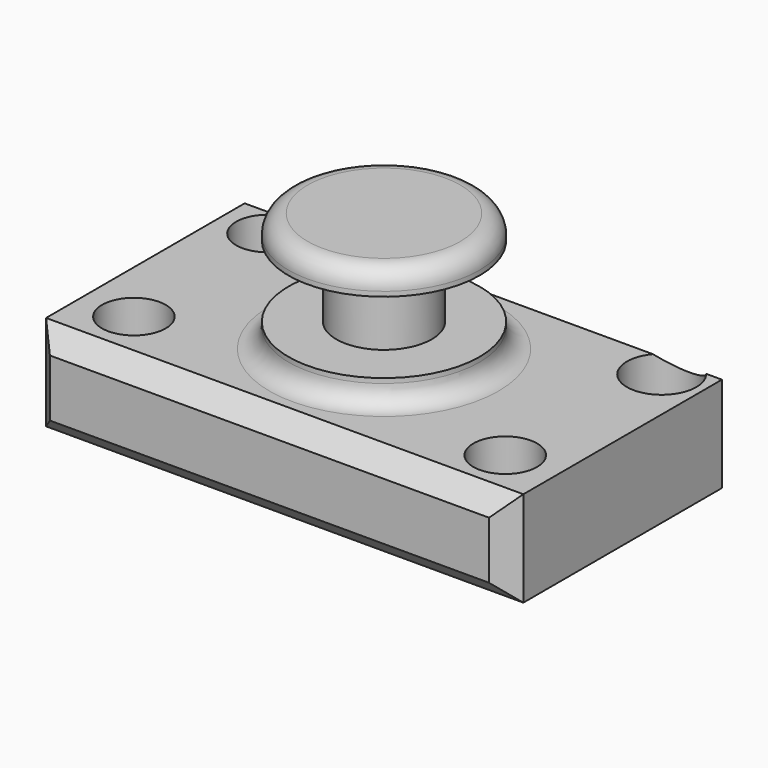
from build123d import *

# Parameters (mm, degrees)
F0_W         = 127
F0_H         = 76.2
F1_DEPTH     = 25.4
F2_R         = 8.4769821521
F2_R_2       = 9.2372123091
F3_DEPTH     = 25.401
F4_W         = 12.7
F4_H         = 25.4
F6_W         = 25.4
F6_H         = 6.35
F8_W         = 25.4
F8_H         = 6.35
F10_R        = 5.08
F11_T1_DEPTH = 51.5282991577
F11_T3_DEPTH = 153.1282991577


# Not quite as in the source:
# - a fillet or chamfer that OpenCascade refuses, or shapes differently, is made with other operations: its cross-section is extruded or revolved along the edge and cut away or added


with BuildPart() as f1:
    # F0 (on Top) → F1 (new body)
    with BuildSketch(Plane.XY):
        Rectangle(F0_W, F0_H)
    extrude(amount=F1_DEPTH)

    # F2 (on face) → F3 (cut, through all)
    with BuildSketch(Plane.XY.offset(25.4)):
        with Locations((-51.2244440438, 25.4412265494)):
            Circle(F2_R)
        with Locations((-49.6174134314, -21.1683232337)):
            Circle(F2_R)
        with Locations((52.2232688963, 27.0741768181)):
            Circle(F2_R_2)
        with Locations((49.5918877423, -21.6549038887)):
            Circle(F2_R)
    extrude(amount=-F3_DEPTH, mode=Mode.SUBTRACT)

    # F4 (on Front) → F5 (revolve)
    with BuildSketch(Plane.XZ):
        with Locations((6.35, 38.1)):
            Rectangle(F4_W, F4_H)
    revolve(axis=Axis((0, 0, 38.1), (0, 0, 1)))

    # F6 (on Front) → F7 (revolve)
    with BuildSketch(Plane.XZ):
        with Locations((12.7, 53.975)):
            Rectangle(F6_W, F6_H)
    revolve(axis=Axis((0, 0, 53.975), (0, 0, -1)))

    # F8 (on Front) → F9 (revolve)
    with BuildSketch(Plane.XZ):
        with Locations((12.7, 28.575)):
            Rectangle(F8_W, F8_H)
    revolve(axis=Axis((0, 0, 28.575), (0, 0, -1)))

    # F10
    f10_edges = [f1.edges().sort_by_distance(p)[0] for p in [
        (-25.4, 0, 57.15),
        (-25.4, 0, 25.4),
    ]]
    fillet(f10_edges, radius=F10_R)

    # F11: chamfer of 5.08 on 8 edges, made by hand

    # F11_s2 → F11_t1 (cut)
    with BuildSketch(Plane.XY.offset(-13.0641495789)):
        Polygon((-58.42, -38.1), (-63.5, -33.02), (-63.5, -38.1), align=None)
        Polygon((63.5, -33.02), (58.42, -38.1), (63.5, -38.1), align=None)
        Polygon((63.5, 33.02), (58.42, 38.1), (63.5, 38.1), align=None)
        Polygon((-58.42, 38.1), (-63.5, 33.02), (-63.5, 38.1), align=None)
    extrude(amount=F11_T1_DEPTH, mode=Mode.SUBTRACT)

    # F11_s4 → F11_t3 (cut)
    with BuildSketch(Plane.YZ.offset(-76.5641495789)):
        Polygon((-38.1, 5.08), (-33.02, 0), (-38.1, 0), align=None)
        Polygon((-33.02, 25.4), (-38.1, 20.32), (-38.1, 25.4), align=None)
        Polygon((38.1, 5.08), (33.02, 0), (38.1, 0), align=None)
        Polygon((33.02, 25.4), (38.1, 20.32), (38.1, 25.4), align=None)
    extrude(amount=F11_T3_DEPTH, mode=Mode.SUBTRACT)


solid = f1.part
